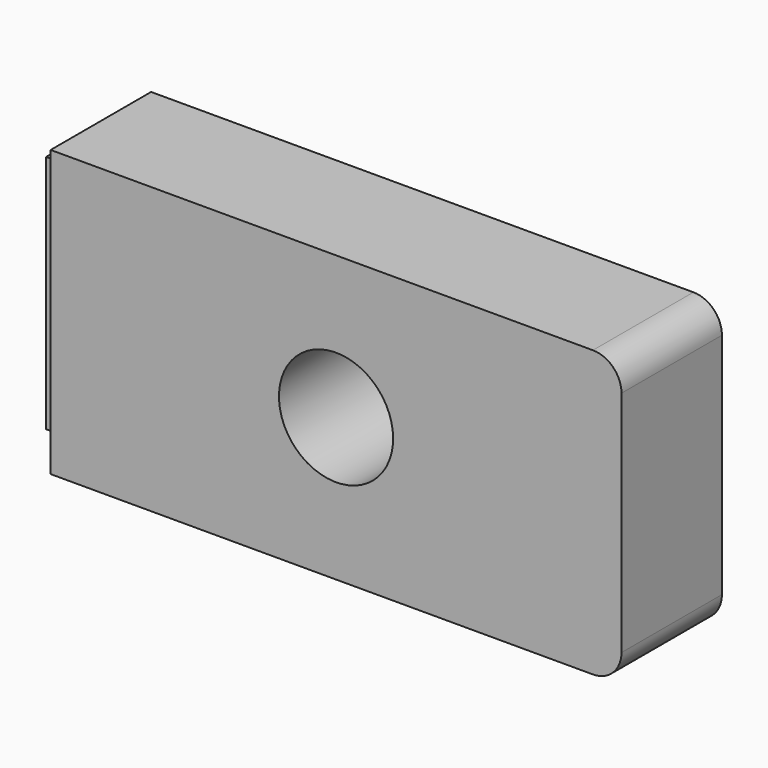
from build123d import *

# Parameters (mm, degrees)
F0_R      = 10
F1_DEPTH  = 20
F1_FACE_R = 10
F2_DEPTH  = 2
F3_W      = 14
F3_H      = 42
F4_DEPTH  = 4


# Not quite as in the source:
# - the program builds the solid bodies; features that only make, move or delete a surface that nothing else refers to are left out


with BuildPart() as f1:
    # F0 (on Front) → F1 (new body)
    with BuildSketch(Plane.XZ):
        with BuildLine():
            Line((45, 25), (-50, 25))
            Line((-50, 25), (-50, -25))
            Line((-50, -25), (45, -25))
            ThreePointArc((45, -25), (48.5355339059, -23.5355339059), (50, -20))
            Line((50, -20), (50, 20))
            ThreePointArc((50, 20), (48.5355339059, 23.5355339059), (45, 25))
        make_face()
        Circle(F0_R, mode=Mode.SUBTRACT)
    extrude(amount=F1_DEPTH)

    # F0 (on Front) + F1_face (on face) → F2 (join)
    with BuildSketch(Plane.XZ):
        with BuildLine():
            Line((45, 25), (-50, 25))
            Line((-50, 25), (-50, -25))
            Line((-50, -25), (45, -25))
            ThreePointArc((45, -25), (48.5355339059, -23.5355339059), (50, -20))
            Line((50, -20), (50, 20))
            ThreePointArc((50, 20), (48.5355339059, 23.5355339059), (45, 25))
        make_face()
        Circle(F0_R, mode=Mode.SUBTRACT)
    with BuildSketch(Plane(origin=(-0.1121943071, -20, 0), x_dir=(1, 0, 0), z_dir=(0, -1, 0))):
        with BuildLine():
            Line((45.1121943071, 25), (-49.8878056929, 25))
            Line((-49.8878056929, 25), (-49.8878056929, -25))
            Line((-49.8878056929, -25), (45.1121943071, -25))
            ThreePointArc((45.1121943071, -25), (48.647728213, -23.5355339059), (50.1121943071, -20))
            Line((50.1121943071, -20), (50.1121943071, 20))
            ThreePointArc((50.1121943071, 20), (48.647728213, 23.5355339059), (45.1121943071, 25))
        make_face()
        with Locations((0.1121943071, 0)):
            Circle(F1_FACE_R, mode=Mode.SUBTRACT)
    extrude(amount=F2_DEPTH)

    # F3 (on face) → F4 (join)
    with BuildSketch(Plane(origin=(-50, 0, 0), x_dir=(0, -1, 0), z_dir=(-1, 0, 0))):
        with Locations((11, 0)):
            Rectangle(F3_W, F3_H)
    extrude(amount=F4_DEPTH)


solid = f1.part
